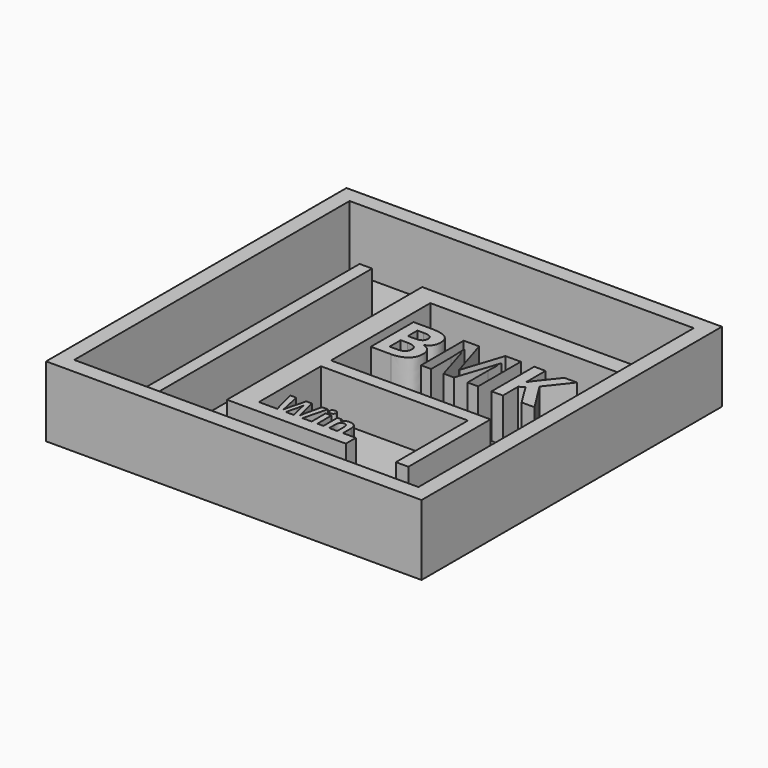
from build123d import *

# Parameters (mm, degrees)
F0_W          = 38.1
F0_H          = 38.1
F1_DEPTH      = 0.79375
F2_W          = 38.1
F2_H          = 38.1
F2_W_2        = 34.925
F2_H_2        = 34.925
F3_DEPTH      = 6.35
F4_W          = 1.27
F4_H          = 29.845
F5_DEPTH      = 4.445
F6_R          = 1.27
F7_DEPTH      = 0.396875
F8_W          = 1.27
F8_H          = 9.1426198413
F8_TEXT_SIZE  = 7.5866391093
F9_DEPTH      = 4.445
F10_R         = 1.27
F11_DEPTH     = 0.4064
F12_TEXT_SIZE = 3.9327005248
F13_DEPTH     = 4.445


# Not quite as in the source:
# - Text() gives the source's letters only with a copy of the font that has no kerning and outlines rounded to 1/6400 em; it was checked with that copy


with BuildPart() as f1:
    # F0 (on Top) → F1 (new body)
    with BuildSketch(Plane.XY):
        with Locations((-1.2958534062, 8.1955464288)):
            Rectangle(F0_W, F0_H)
    extrude(amount=F1_DEPTH)

    # F2 (on face) → F3 (join)
    with BuildSketch(Plane.XY.offset(0.79375)):
        with Locations((-1.2958534062, 8.1955464288)):
            Rectangle(F2_W, F2_H)
        with Locations((-1.2958534062, 8.1955464288)):
            Rectangle(F2_W_2, F2_H_2, mode=Mode.SUBTRACT)
    extrude(amount=F3_DEPTH)

    # F4 (on face) → F5 (join)
    with BuildSketch(Plane.XY.offset(0.79375)):
        with Locations((-13.0433534062, 5.6555464288)):
            Rectangle(F4_W, F4_H)
    extrude(amount=F5_DEPTH)

    # F6 (on face) → F7 (cut)
    with BuildSketch(Plane.XY.offset(0.79375)):
        with Locations((-16.2183534062, -7.2972238995)):
            Circle(F6_R)
    extrude(amount=-F7_DEPTH, mode=Mode.SUBTRACT)

    # F8 (on face) → F9 (join)
    with BuildSketch(Plane.XY.offset(0.79375)):
        Polygon((-3.3610837954, 20.5780464288), (-7.3283534062, 20.5780464288), (-7.3283534062, 18.8279598951), (-7.3283534062, 4.9556662702), (-7.3283534062, -4.1869535712), (-5.1029655647, -4.1869535712), (4.7366465938, -4.1869535712), (4.7366465938, -2.9169535712), (-5.1029655647, -2.9169535712), (-5.1029655647, 4.9556662702), (-5.1029655647, 6.2256662702), (-5.1029655647, 18.8279598951), (16.1666465938, 18.8279598951), (16.1666465938, 20.5780464288), (10.0829654184, 20.5780464288), (7.9399986935, 20.5780464288), (-2.0330404586, 20.5780464288), align=None)
        Polygon((11.0866465938, 6.2256662702), (-5.1029655647, 6.2256662702), (-5.1029655647, 4.9556662702), (-0.0294123298, 4.9556662702), (2.6080856346, 4.9556662702), (9.8166465938, 4.9556662702), (11.0866465938, 4.9556662702), align=None)
        with Locations((10.4516465938, 0.3843563495)):
            Rectangle(F8_W, F8_H)
        with Locations((-4.7883534062, 10.0356662702)):
            Text('BMK', F8_TEXT_SIZE, font='Open Sans', font_style=FontStyle.BOLD, text_align=(TextAlign.LEFT, TextAlign.BOTTOM))
    extrude(amount=F9_DEPTH)

    # F10 (on face) → F11 (cut)
    with BuildSketch(Plane.XY.offset(0.79375)):
        with Locations((-2.1328919102, 2.1903254092)):
            Circle(F10_R)
    extrude(amount=-F11_DEPTH, mode=Mode.SUBTRACT)

    # F12 (on face) → F13 (join)
    with BuildSketch(Plane.XY.offset(0.79375)):
        with Locations((-3.8637830876, -3.2870387658)):
            Text('Win', F12_TEXT_SIZE, font='Open Sans', font_style=FontStyle.BOLD, text_align=(TextAlign.LEFT, TextAlign.BOTTOM))
    extrude(amount=F13_DEPTH)


solid = f1.part
